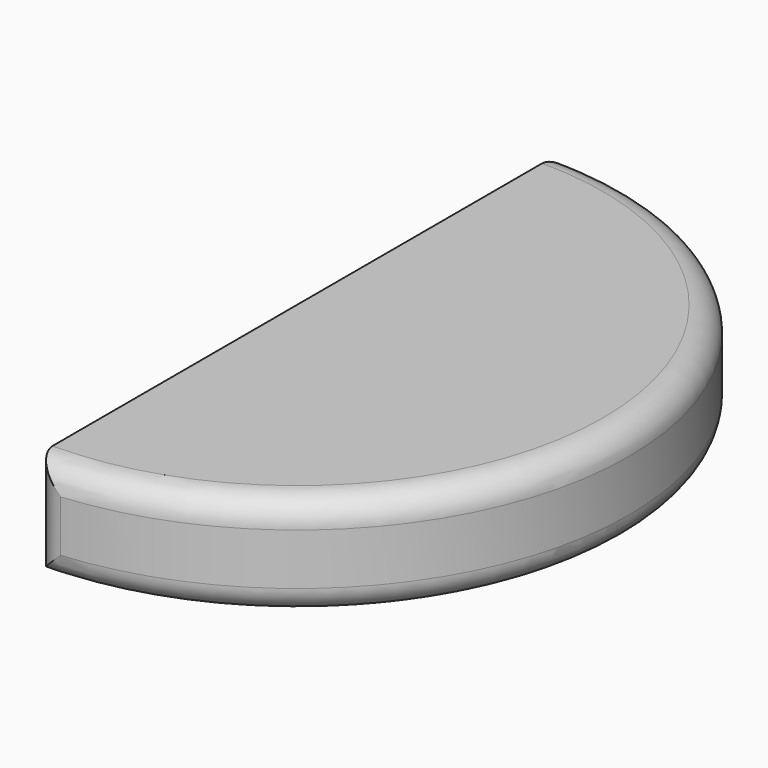
from build123d import *

# Parameters (mm, degrees)
F1_DEPTH = 203.2
F2_R     = 50.8


with BuildPart() as f1:
    # F0 (on Top) → F1 (new body)
    with BuildSketch(Plane.XY):
        with BuildLine():
            ThreePointArc((0, -654.99996), (654.99996, 0), (0, 654.99996))
            Line((0, 654.99996), (0, -654.99996))
        make_face()
    extrude(amount=F1_DEPTH)

    # F2
    f2_edges = [f1.edges().sort_by_distance(p)[0] for p in [
        (654.99996, 0, 203.2),
        (654.99996, 0, 0),
        (0, 654.99996, 101.6),
        (0, -654.99996, 101.6),
    ]]
    fillet(f2_edges, radius=F2_R)


solid = f1.part
